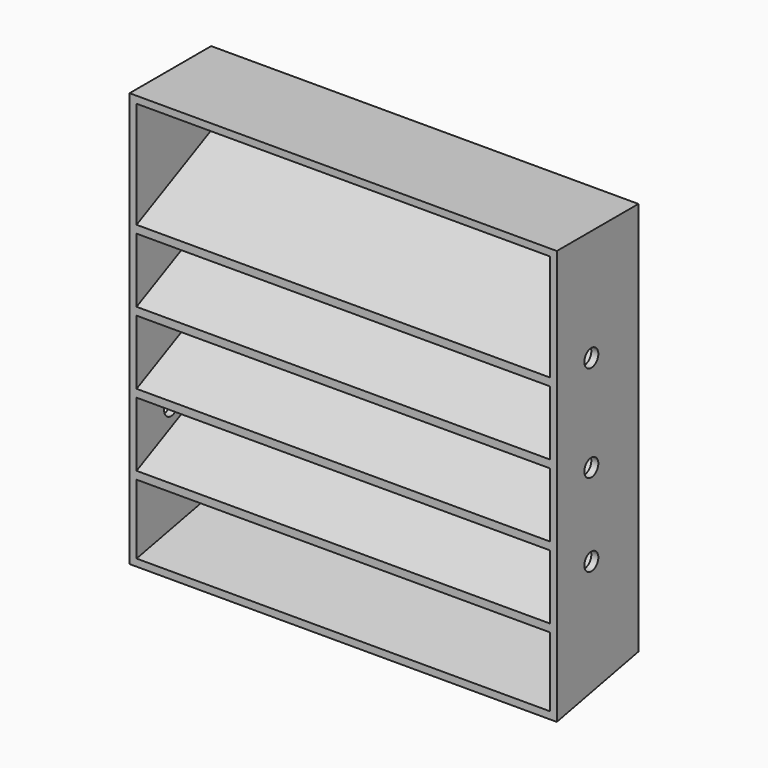
from build123d import *

# Parameters (mm, degrees)
F0_W        = 155
F0_H        = 151
F1_DEPTH    = 37
F2_T1_DEPTH = 362.8505669038
F3_T        = -2.54
F4_W        = 125.55387271
F4_H        = 111.9176980871
F5_DEPTH    = 25.4
F6_R        = 3.175
F7_DEPTH    = 155.001
F9_DEPTH    = 152.46


# Not quite as in the source:
# - a fillet or chamfer that OpenCascade refuses, or shapes differently, is made with other operations: its cross-section is extruded or revolved along the edge and cut away or added


with BuildPart() as f1:
    # F0 (on Front) → F1 (new body)
    with BuildSketch(Plane.XZ):
        Rectangle(F0_W, F0_H)
    extrude(amount=F1_DEPTH)

    # F2: chamfer of 40 x 8 on 1 edges, made by hand

    # F2_s2 → F2_t1 (cut)
    with BuildSketch(Plane.YZ.offset(-181.4252834519)):
        Polygon((-40, -75.5), (0, -67.5), (0, -75.5), align=None)
    extrude(amount=F2_T1_DEPTH, mode=Mode.SUBTRACT)

    # F3
    f3_openings = [f1.faces().sort_by_distance(p)[0] for p in [
        (0, -37, 0.3),
    ]]
    offset(amount=F3_T, openings=f3_openings)

    # F4 (on face) → F5 (cut)
    with BuildSketch(Plane.XZ.offset(2.54)):
        with Locations((-0.276936355, 9.5411509565)):
            Rectangle(F4_W, F4_H)
    extrude(amount=-F5_DEPTH, mode=Mode.SUBTRACT)

    # F6 (on face) → F7 (cut, through all)
    with BuildSketch(Plane(origin=(-77.5, 0, 0), x_dir=(0, -1, 0), z_dir=(-1, 0, 0))):
        with Locations((21.3561020792, 0)):
            Circle(F6_R)
        with Locations((21.3561020792, 35)):
            Circle(F6_R)
        with Locations((21.3561020792, -30)):
            Circle(F6_R)
    extrude(amount=-F7_DEPTH, mode=Mode.SUBTRACT)

    # F8 (on face) → F9 (join, through all)
    with BuildSketch(Plane(origin=(74.96, 0, 0), x_dir=(0, -1, 0), z_dir=(-1, 0, 0))):
        Polygon((0, -29.1507557497), (37, -47.1048012634), (37, -44.281557044), (0, -26.3275115302), align=None)
        Polygon((0, -2.9595115302), (37, -20.913557044), (37, -18.0903128246), (0, -0.1362673108), align=None)
        Polygon((0, 23.2317326892), (37, 5.2776871754), (37, 8.1009313948), (0, 26.0549769086), align=None)
        Polygon((0, 49.4229769086), (37, 31.4689313948), (37, 34.2921756143), (0, 52.246221128), align=None)
    extrude(amount=F9_DEPTH)


solid = f1.part
